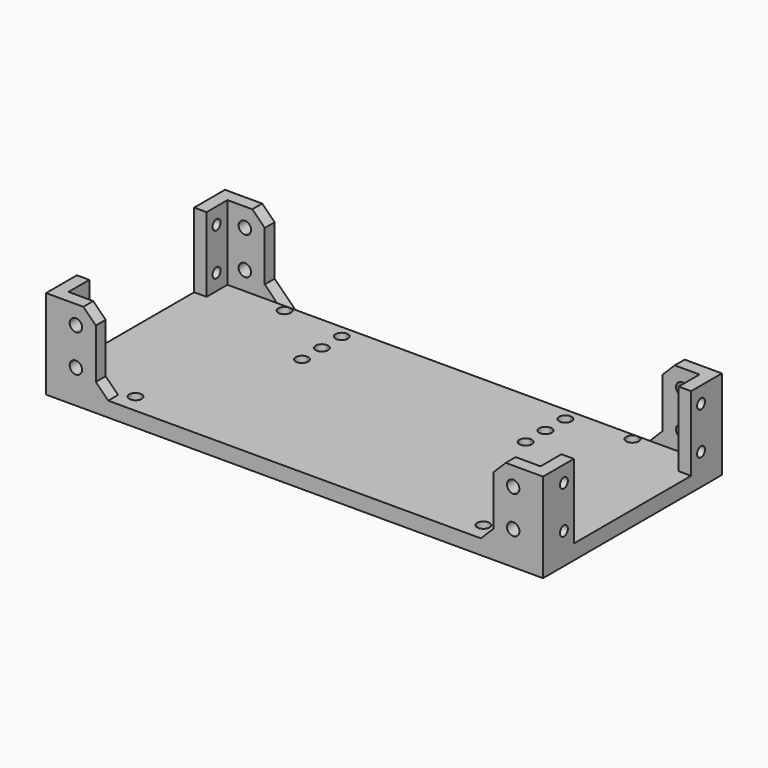
from build123d import *

# Parameters (mm, degrees)
F1_DEPTH = 6
F2_DEPTH = 36
F3_SIZE  = 5
F6_DEPTH = 210
F7_DEPTH = 100
F8_SIZE  = 4.99999


# Not quite as in the source:
# - a fillet or chamfer is up to 0.001 mm smaller than in the source, because OpenCascade refuses the exact size


with BuildPart() as f1:
    # F0 (on Top) → F1 (new body)
    with BuildSketch(Plane.XY):
        with BuildLine():
            Line((20, 5), (20, 0))
            Line((20, 0), (30, 0))
            Line((30, 0), (170, 0))
            Line((170, 0), (180, 0))
            Line((180, 0), (180, 5))
            Line((180, 5), (195, 5))
            Line((195, 5), (195, 15.5))
            Line((195, 15.5), (200, 15.5))
            Line((200, 15.5), (200, 74.5))
            Line((200, 74.5), (195, 74.5))
            Line((195, 74.5), (195, 85))
            Line((195, 85), (180, 85))
            Line((180, 85), (180, 90))
            Line((180, 90), (170, 90))
            Line((170, 90), (145, 90))
            Line((145, 90), (145, 82.5))
            ThreePointArc((145, 82.5), (146.767766953, 81.767766953), (147.5, 80))
            ThreePointArc((147.5, 80), (146.767766953, 78.232233047), (145, 77.5))
            Line((145, 77.5), (145, 72.5))
            ThreePointArc((145, 72.5), (146.767766953, 71.767766953), (147.5, 70))
            ThreePointArc((147.5, 70), (146.767766953, 68.232233047), (145, 67.5))
            Line((145, 67.5), (145, 62.5))
            ThreePointArc((145, 62.5), (146.767766953, 61.767766953), (147.5, 60))
            ThreePointArc((147.5, 60), (145, 57.5), (142.5, 60))
            Line((142.5, 60), (100, 60))
            Line((100, 60), (57.5, 60))
            ThreePointArc((57.5, 60), (53.232233047, 58.232233047), (55, 62.5))
            Line((55, 62.5), (55, 67.5))
            ThreePointArc((55, 67.5), (52.5, 70), (55, 72.5))
            Line((55, 72.5), (55, 77.5))
            ThreePointArc((55, 77.5), (52.5, 80), (55, 82.5))
            Line((55, 82.5), (55, 90))
            Line((55, 90), (30, 90))
            Line((30, 90), (20, 90))
            Line((20, 90), (20, 85))
            Line((20, 85), (5, 85))
            Line((5, 85), (5, 74.5))
            Line((5, 74.5), (0, 74.5))
            Line((0, 74.5), (0, 15.5))
            Line((0, 15.5), (5, 15.5))
            Line((5, 15.5), (5, 5))
            Line((5, 5), (20, 5))
        make_face()
        with BuildLine():
            ThreePointArc((32.5, 7.5), (31.767766953, 5.732233047), (30, 5))
            ThreePointArc((30, 5), (28.232233047, 9.267766953), (32.5, 7.5))
        make_face(mode=Mode.SUBTRACT)
        with BuildLine():
            ThreePointArc((172.5, 7.5), (171.767766953, 5.732233047), (170, 5))
            ThreePointArc((170, 5), (168.232233047, 9.267766953), (172.5, 7.5))
        make_face(mode=Mode.SUBTRACT)
        with BuildLine():
            ThreePointArc((32.5, 82.5), (28.232233047, 80.732233047), (30, 85))
            ThreePointArc((30, 85), (31.767766953, 84.267766953), (32.5, 82.5))
        make_face(mode=Mode.SUBTRACT)
        with BuildLine():
            ThreePointArc((172.5, 82.5), (168.232233047, 80.732233047), (170, 85))
            ThreePointArc((170, 85), (171.767766953, 84.267766953), (172.5, 82.5))
        make_face(mode=Mode.SUBTRACT)
        with BuildLine():
            Line((100, 90), (55, 90))
            Line((55, 90), (55, 82.5))
            ThreePointArc((55, 82.5), (56.767766953, 81.767766953), (57.5, 80))
            ThreePointArc((57.5, 80), (56.767766953, 78.232233047), (55, 77.5))
            Line((55, 77.5), (55, 72.5))
            ThreePointArc((55, 72.5), (56.767766953, 71.767766953), (57.5, 70))
            ThreePointArc((57.5, 70), (56.767766953, 68.232233047), (55, 67.5))
            Line((55, 67.5), (55, 62.5))
            ThreePointArc((55, 62.5), (56.767766953, 61.767766953), (57.5, 60))
            Line((57.5, 60), (100, 60))
            Line((100, 60), (100, 90))
        make_face()
        with BuildLine():
            Line((145, 90), (100, 90))
            Line((100, 90), (100, 60))
            Line((100, 60), (142.5, 60))
            ThreePointArc((142.5, 60), (143.232233047, 61.767766953), (145, 62.5))
            Line((145, 62.5), (145, 67.5))
            ThreePointArc((145, 67.5), (142.5, 70), (145, 72.5))
            Line((145, 72.5), (145, 77.5))
            ThreePointArc((145, 77.5), (142.5, 80), (145, 82.5))
            Line((145, 82.5), (145, 90))
        make_face()
    extrude(amount=F1_DEPTH)

    # F0 (on Top) → F2 (join)
    with BuildSketch(Plane.XY):
        Polygon((195, 74.5), (200, 74.5), (200, 90), (180, 90), (180, 85), (195, 85), align=None)
        Polygon((180, 5), (180, 0), (200, 0), (200, 15.5), (195, 15.5), (195, 5), align=None)
        Polygon((0, 15.5), (0, 0), (20, 0), (20, 5), (5, 5), (5, 15.5), align=None)
        Polygon((0, 90), (0, 74.5), (5, 74.5), (5, 85), (20, 85), (20, 90), align=None)
    extrude(amount=F2_DEPTH)

    # F3
    f3_edges = [f1.edges().sort_by_distance(p)[0] for p in [
        (180, 87.5, 6),
        (180, 2.5, 6),
        (180, 2.5, 36),
        (180, 87.5, 36),
        (20, 87.5, 36),
        (20, 2.5, 36),
        (20, 87.5, 6),
        (20, 2.5, 6),
    ]]
    chamfer(f3_edges, length=F3_SIZE)

    # F5 (on face) → F6 (cut)
    with BuildSketch(Plane(origin=(0, 0, 0), x_dir=(0, -1, 0), z_dir=(-1, 0, 0))):
        with BuildLine():
            ThreePointArc((-77.5, 29.5), (-80.9142135624, 30.9142135624), (-79.5, 27.5))
            ThreePointArc((-79.5, 27.5), (-78.0857864376, 28.0857864376), (-77.5, 29.5))
        make_face()
        with BuildLine():
            ThreePointArc((-77.5, 12.5), (-78.0857864376, 13.9142135624), (-79.5, 14.5))
            ThreePointArc((-79.5, 14.5), (-80.9142135624, 11.0857864376), (-77.5, 12.5))
        make_face()
        with BuildLine():
            ThreePointArc((-8.5, 29.5), (-11.9142135624, 30.9142135624), (-10.5, 27.5))
            ThreePointArc((-10.5, 27.5), (-9.0857864376, 28.0857864376), (-8.5, 29.5))
        make_face()
        with BuildLine():
            ThreePointArc((-8.5, 12.5), (-9.0857864376, 13.9142135624), (-10.5, 14.5))
            ThreePointArc((-10.5, 14.5), (-11.9142135624, 11.0857864376), (-8.5, 12.5))
        make_face()
    extrude(amount=-F6_DEPTH, mode=Mode.SUBTRACT)

    # F4 (on face) → F7 (cut)
    with BuildSketch(Plane.XZ):
        with BuildLine():
            ThreePointArc((14.5, 28.5), (10.232233047, 30.267766953), (12, 26))
            ThreePointArc((12, 26), (13.767766953, 26.732233047), (14.5, 28.5))
        make_face()
        with BuildLine():
            ThreePointArc((14.5, 13.5), (13.767766953, 15.267766953), (12, 16))
            ThreePointArc((12, 16), (10.232233047, 11.732233047), (14.5, 13.5))
        make_face()
        with BuildLine():
            ThreePointArc((190.5, 28.5), (186.232233047, 30.267766953), (188, 26))
            ThreePointArc((188, 26), (189.767766953, 26.732233047), (190.5, 28.5))
        make_face()
        with BuildLine():
            ThreePointArc((190.5, 13.5), (189.767766953, 15.267766953), (188, 16))
            ThreePointArc((188, 16), (186.232233047, 11.732233047), (190.5, 13.5))
        make_face()
    extrude(amount=-F7_DEPTH, mode=Mode.SUBTRACT)

    # F8 (size 5 in the source; OpenCascade refuses exactly that, so slightly less here)
    f8_edges = [f1.edges().sort_by_distance(p)[0] for p in [
        (100, 90, 6),
    ]]
    chamfer(f8_edges, length=F8_SIZE)


solid = f1.part
